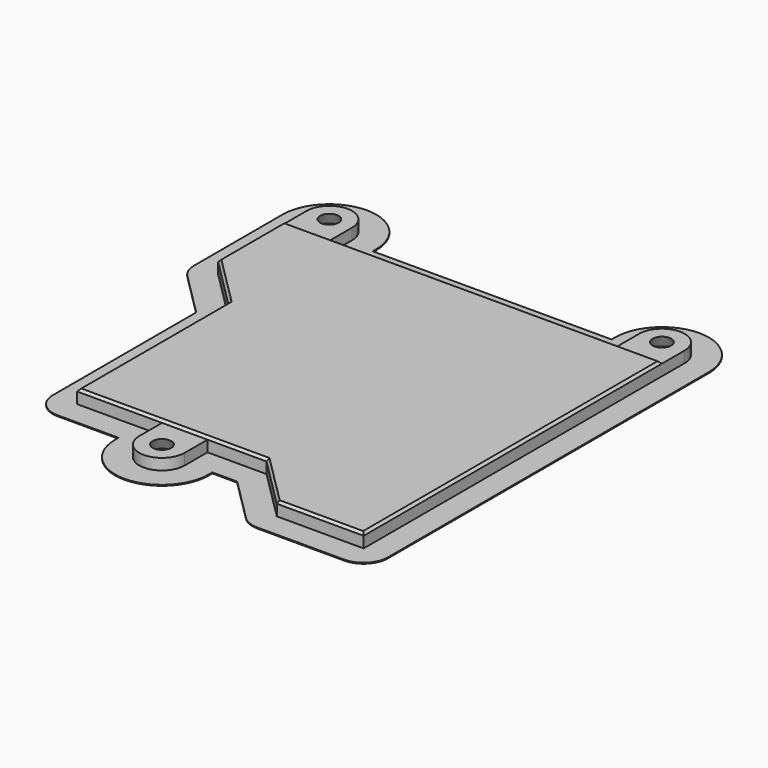
from build123d import *

# Parameters (mm, degrees)
F0_R     = 1.75
F1_DEPTH = 3
F2_SIZE2 = 2.8
F2_SIZE  = 1.6
F4_DEPTH = 0.5
F5_SIZE  = 0.49999
F7_DEPTH = 0.2


# Not quite as in the source:
# - a fillet or chamfer is up to 0.001 mm smaller than in the source, because OpenCascade refuses the exact size


with BuildPart() as f1:
    # F0 (on Top) → F1 (new body)
    with BuildSketch(Plane.XY):
        with BuildLine():
            Line((18.2, -38.893), (18.2, -44.793))
            ThreePointArc((18.2, -44.793), (22.9, -49.493), (27.6, -44.793))
            Line((27.6, -44.793), (27.6, -38.893))
            Line((27.6, -38.893), (39.8048274606, -38.893))
            Line((39.8048274606, -38.893), (50.3215900894, -49.3928583233))
            Line((50.3215900894, -49.3928583233), (68.3003446043, -49.3928583233))
            Line((68.3003446043, -49.3928583233), (68.3003446043, 33.6071416767))
            ThreePointArc((68.3003446043, 33.6071416767), (63.6003446043, 38.3071416767), (58.9003446043, 33.6071416767))
            Line((58.9003446043, 33.6071416767), (58.9003446043, 27.7071416767))
            Line((58.9003446043, 27.7071416767), (-0.4976553957, 27.7071416767))
            Line((-0.4976553957, 27.7071416767), (-0.4976553957, 33.6071416767))
            ThreePointArc((-0.4976553957, 33.6071416767), (-5.1976553957, 38.3071416767), (-9.8976553957, 33.6071416767))
            Line((-9.8976553957, 33.6071416767), (-9.8976553957, 10.7295926865))
            Line((-9.8976553957, 10.7295926865), (0.6, 0.248810884))
            Line((0.6, 0.248810884), (0.6, -38.893))
            Line((0.6, -38.893), (18.2, -38.893))
        make_face()
        with Locations((22.9, -44.793)):
            Circle(F0_R, mode=Mode.SUBTRACT)
        with Locations((-5.1976553957, 33.6071416767)):
            Circle(F0_R, mode=Mode.SUBTRACT)
        with Locations((63.6003446043, 33.6071416767)):
            Circle(F0_R, mode=Mode.SUBTRACT)
    extrude(amount=F1_DEPTH)

    # F2
    f2_edges = [f1.edges().sort_by_distance(p)[0] for p in [
        (21.15, -44.793, 0),
        (-6.947655, 33.607142, 0),
        (61.850345, 33.607142, 0),
    ]]
    f2_side = f1.faces().sort_by_distance((33.412828, -5.806914, 0))[0]
    chamfer(f2_edges, length=F2_SIZE, length2=F2_SIZE2, reference=f2_side)

    # F3 (on face) → F4 (cut)
    with BuildSketch(Plane.XY.offset(3)):
        with BuildLine():
            Line((-9.8976553957, 27.7071416767), (-0.4976553957, 27.7071416767))
            Line((-0.4976553957, 27.7071416767), (-0.4976553957, 33.6071416767))
            ThreePointArc((-0.4976553957, 33.6071416767), (-5.1976553957, 38.3071416767), (-9.8976553957, 33.6071416767))
            Line((-9.8976553957, 33.6071416767), (-9.8976553957, 27.7071416767))
        make_face()
        with BuildLine():
            Line((58.9003446043, 33.6071416767), (58.9003446043, 27.7071416767))
            Line((58.9003446043, 27.7071416767), (68.3003446043, 27.7071416767))
            Line((68.3003446043, 27.7071416767), (68.3003446043, 33.6071416767))
            ThreePointArc((68.3003446043, 33.6071416767), (63.6003446043, 38.3071416767), (58.9003446043, 33.6071416767))
        make_face()
        with BuildLine():
            Line((27.6, -38.893), (18.2, -38.893))
            Line((18.2, -38.893), (18.2, -44.793))
            ThreePointArc((18.2, -44.793), (22.9, -49.493), (27.6, -44.793))
            Line((27.6, -44.793), (27.6, -38.893))
        make_face()
    extrude(amount=-F4_DEPTH, mode=Mode.SUBTRACT)

    # F5 (size 0.5 in the source; OpenCascade refuses exactly that, so slightly less here)
    f5_edges = [f1.edges().sort_by_distance(p)[0] for p in [
        (29.201345, 27.707142, 3),
        (-9.897655, 19.218367, 3),
        (-4.648828, 5.489202, 3),
        (0.6, -19.322095, 3),
        (20.202414, -38.893, 3),
        (45.063209, -44.142929, 3),
        (59.310967, -49.392858, 3),
        (68.300345, -10.842858, 3),
    ]]
    chamfer(f5_edges, length=F5_SIZE)

    # F6 (on face) → F7 (join)
    with BuildSketch(Plane(origin=(0, 0, 0), x_dir=(1, 0, 0), z_dir=(0, 0, -1))):
        with BuildLine():
            ThreePointArc((0.6, 43.893), (-2.9355339059, 42.4285339059), (-4.4, 38.893))
            Line((-4.4, 38.893), (-4.4, 1.824613149))
            Line((-4.4, 1.824613149), (-13.4303444218, -7.1912161881))
            ThreePointArc((-13.4303444218, -7.1912161881), (-14.5162831751, -8.8143179191), (-14.8976553957, -10.7295926865))
            Line((-14.8976553957, -10.7295926865), (-14.8976553957, -33.6071416767))
            ThreePointArc((-14.8976553957, -33.6071416767), (-5.1976553957, -43.3071416767), (4.5023446043, -33.6071416767))
            Line((4.5023446043, -33.6071416767), (4.5023446043, -32.7071416767))
            Line((4.5023446043, -32.7071416767), (53.9003446043, -32.7071416767))
            Line((53.9003446043, -32.7071416767), (53.9003446043, -33.6071416767))
            ThreePointArc((53.9003446043, -33.6071416767), (63.6003446043, -43.3071416767), (73.3003446043, -33.6071416767))
            Line((73.3003446043, -33.6071416767), (73.3003446043, 49.3928583233))
            ThreePointArc((73.3003446043, 49.3928583233), (71.8358785102, 52.9283922293), (68.3003446043, 54.3928583233))
            Line((68.3003446043, 54.3928583233), (50.3215900894, 54.3928583233))
            ThreePointArc((50.3215900894, 54.3928583233), (48.4100308427, 54.0130251219), (46.7889010633, 52.9312348218))
            Line((46.7889010633, 52.9312348218), (37.736115085, 43.893))
            Line((37.736115085, 43.893), (32.6, 43.893))
            Line((32.6, 43.893), (32.6, 44.793))
            ThreePointArc((32.6, 44.793), (22.9, 54.493), (13.2, 44.793))
            Line((13.2, 44.793), (13.2, 43.893))
            Line((13.2, 43.893), (0.6, 43.893))
        make_face()
        with BuildLine():
            Line((-9.8976553957, -33.6071416767), (-9.8976553957, -10.7295926865))
            Line((-9.8976553957, -10.7295926865), (0.6, -0.248810884))
            Line((0.6, -0.248810884), (0.6, 38.893))
            Line((0.6, 38.893), (18.2, 38.893))
            Line((18.2, 38.893), (18.2, 44.793))
            ThreePointArc((18.2, 44.793), (22.9, 49.493), (27.6, 44.793))
            Line((27.6, 44.793), (27.6, 38.893))
            Line((27.6, 38.893), (39.8048274606, 38.893))
            Line((39.8048274606, 38.893), (50.3215900894, 49.3928583233))
            Line((50.3215900894, 49.3928583233), (68.3003446043, 49.3928583233))
            Line((68.3003446043, 49.3928583233), (68.3003446043, -33.6071416767))
            ThreePointArc((68.3003446043, -33.6071416767), (63.6003446043, -38.3071416767), (58.9003446043, -33.6071416767))
            Line((58.9003446043, -33.6071416767), (58.9003446043, -27.7071416767))
            Line((58.9003446043, -27.7071416767), (-0.4976553957, -27.7071416767))
            Line((-0.4976553957, -27.7071416767), (-0.4976553957, -33.6071416767))
            ThreePointArc((-0.4976553957, -33.6071416767), (-5.1976553957, -38.3071416767), (-9.8976553957, -33.6071416767))
        make_face(mode=Mode.SUBTRACT)
    extrude(amount=-F7_DEPTH)


solid = f1.part
